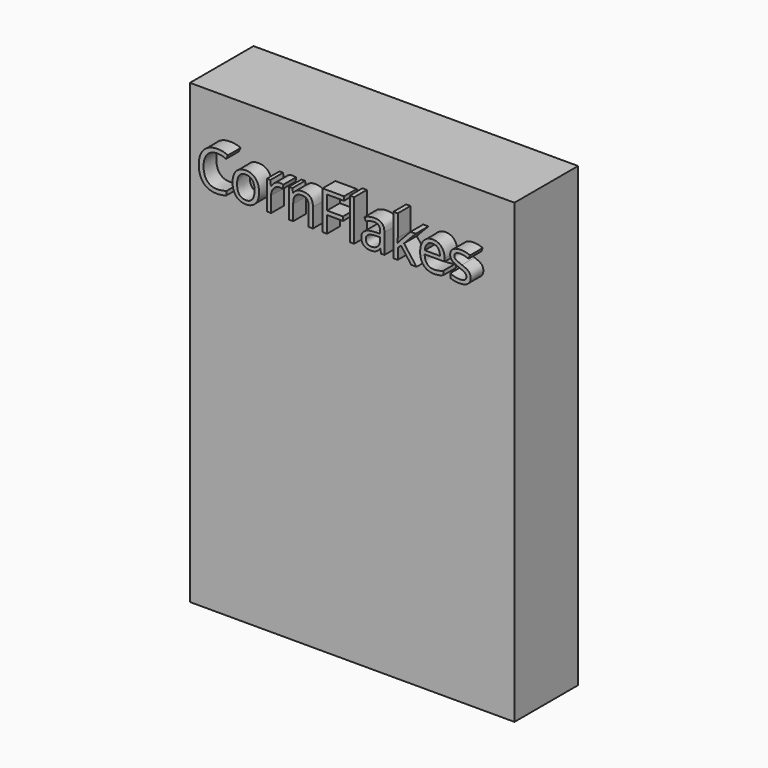
from build123d import *

# Parameters (mm, degrees)
F0_W         = 40.8120448701
F0_H         = 57.4817503802
F1_DEPTH     = 10
F2_TEXT_SIZE = 6.7860405478
F3_DEPTH     = 12


# Not quite as in the source:
# - Text() gives the source's letters only with a copy of the font that has no kerning and outlines rounded to 1/6400 em; it was checked with that copy


with BuildPart() as f1:
    # F0 (on Front) → F1 (new body)
    with BuildSketch(Plane.XZ):
        with Locations((-27.7349466924, 34.9201636855)):
            Rectangle(F0_W, F0_H)
    extrude(amount=F1_DEPTH)

    # F2 (on Front) → F3 (join)
    with BuildSketch(Plane.XZ):
        with Locations((-45.8417022601, 53.8891479373)):
            Text('CornFlakes', F2_TEXT_SIZE, font='Open Sans', text_align=(TextAlign.LEFT, TextAlign.BOTTOM))
    extrude(amount=F3_DEPTH)


solid = f1.part
